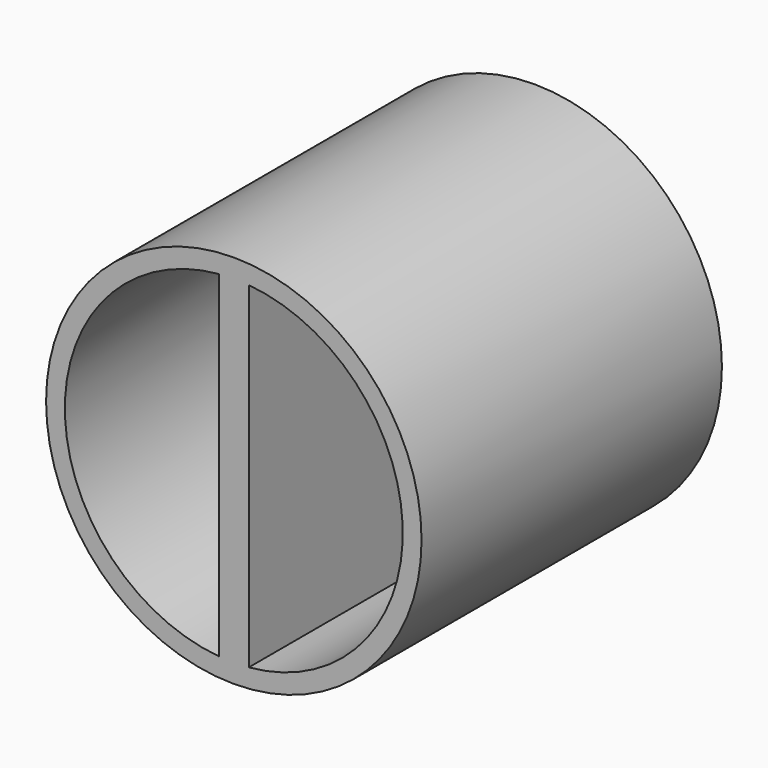
from build123d import *

# Parameters (mm, degrees)
F0_R     = 63.5
F1_DEPTH = 127
F4_D     = 114.3
F5_DEPTH = 25.4
F6_W     = 10.1255085319
F6_H     = 120.7859069109
F7_DEPTH = 101.6


# Not quite as in the source:
# - a feature names something its author has since deleted; it is built from what else it names


with BuildPart() as f1:
    # F0 (on Front) → F1 (new body)
    with BuildSketch(Plane.XZ):
        Circle(F0_R)
    extrude(amount=F1_DEPTH)

    # F4 (through all)
    with Locations(Plane(origin=(0, 0, 0), x_dir=(-1, 0, 0), z_dir=(0, 1, 0))):
        with Locations((0, 0)):
            Hole(F4_D / 2)

    # F0 (on Front) → F5 (join)
    with BuildSketch(Plane.XZ):
        Circle(F0_R)
    extrude(amount=F5_DEPTH)

    # F6 (on face) → F7 (join)
    with BuildSketch(Plane.XZ.offset(25.4)):
        Rectangle(F6_W, F6_H)
    extrude(amount=F7_DEPTH)


solid = f1.part
